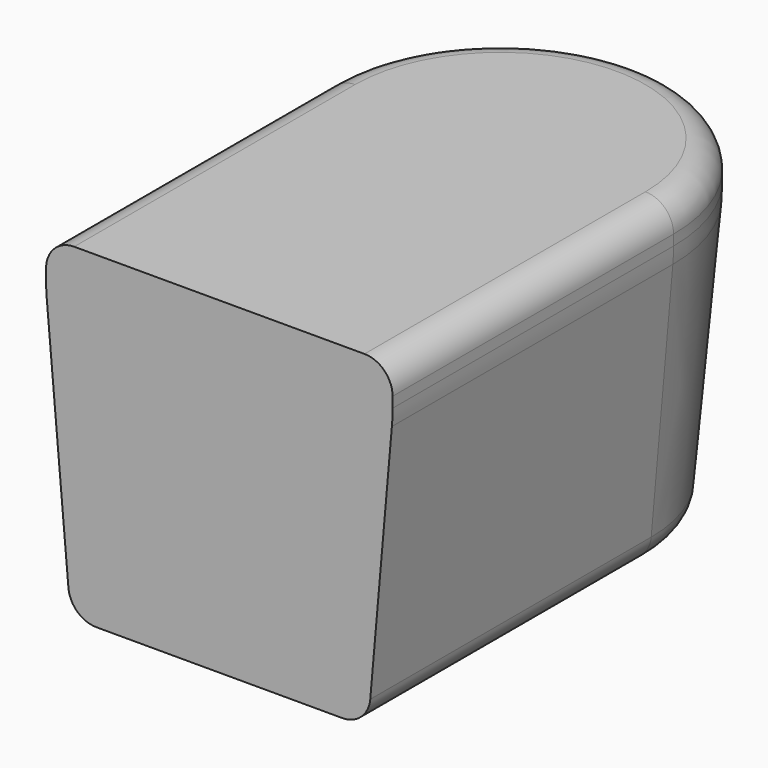
from build123d import *

# Parameters (mm, degrees)
F1_DEPTH    = 350
F2_SIZE2    = 26.2465990578
F2_SIZE     = 300
F3_T1_DEPTH = 396.8304714543
F3_T4_ANGLE = 180
F4_R        = 30


# Not quite as in the source:
# - a fillet or chamfer that OpenCascade refuses, or shapes differently, is made with other operations: its cross-section is extruded or revolved along the edge and cut away or added


with BuildPart() as f1:
    # F0 (on Top) → F1 (new body)
    with BuildSketch(Plane.XY):
        with BuildLine():
            Line((-185, 375), (-185, 0))
            Line((-185, 0), (185, 0))
            Line((185, 0), (185, 375))
            ThreePointArc((185, 375), (130.8147545195, 505.8147545195), (0, 560))
            ThreePointArc((0, 560), (-130.8147545195, 505.8147545195), (-185, 375))
        make_face()
    extrude(amount=F1_DEPTH)

    # F2
    f2_edges = [f1.edges().sort_by_distance(p)[0] for p in [
        (185, 187.5, 0),
        (0, 560, 0),
        (-185, 187.5, 0),
    ]]
    chamfer(f2_edges, length=F2_SIZE, length2=F2_SIZE2)

    # F3: fillet of radius 200 on 3 edges, made by hand

    # F3_s2 → F3_t1 (cut)
    with BuildSketch(Plane.XZ.offset(-375)):
        with BuildLine():
            ThreePointArc((-185, 308.7321885817), (-184.8096443164, 300.0083111086), (-184.2389396183, 291.3010400322))
            Line((-184.2389396183, 291.3010400322), (-185, 300))
            Line((-185, 300), (-185, 308.7321885817))
        make_face()
        with BuildLine():
            ThreePointArc((185, 308.7321885817), (184.8096443164, 300.0083111086), (184.2389396183, 291.3010400322))
            Line((184.2389396183, 291.3010400322), (185, 300))
            Line((185, 300), (185, 308.7321885817))
        make_face()
    extrude(amount=F3_T1_DEPTH, mode=Mode.SUBTRACT)

    # F3_s3 → F3_t4 (revolve, cut)
    with BuildSketch(Plane.XZ.offset(-375)):
        with BuildLine():
            ThreePointArc((185, 308.7321885817), (184.8096443164, 300.0083111086), (184.2389396183, 291.3010400322))
            Line((184.2389396183, 291.3010400322), (185, 300))
            Line((185, 300), (185, 308.7321885817))
        make_face()
    revolve(axis=Axis((0, 375, 300), (0, 0, 1)), revolution_arc=F3_T4_ANGLE, mode=Mode.SUBTRACT)

    # F4
    f4_edges = [f1.edges().sort_by_distance(p)[0] for p in [
        (158.753401, 187.5, 0),
        (0, 533.753401, 0),
        (-158.753401, 187.5, 0),
        (185, 187.5, 350),
        (0, 560, 350),
        (-185, 187.5, 350),
    ]]
    fillet(f4_edges, radius=F4_R)


solid = f1.part
